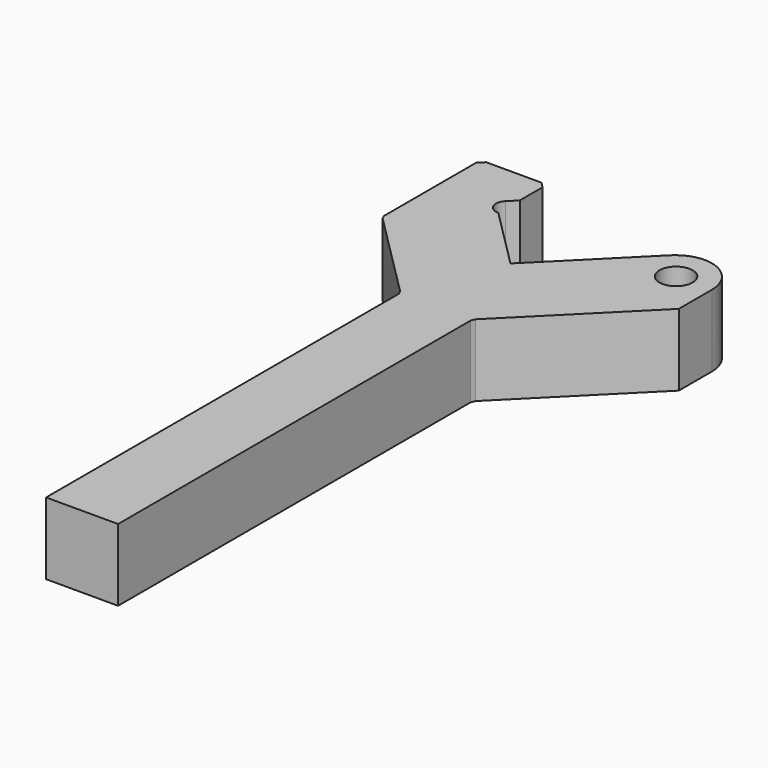
from build123d import *

# Parameters (mm, degrees)
F0_R        = 3
F1_DEPTH    = 13
F2_R        = 7
F3_R        = 6.5
F4_T1_DEPTH = 13
F4_T3_DEPTH = 18.1433659759
F4_T5_DEPTH = 15.2571417204


# Not quite as in the source:
# - a fillet or chamfer that OpenCascade refuses, or shapes differently, is made with other operations: its cross-section is extruded or revolved along the edge and cut away or added


with BuildPart() as f1:
    # F0 (on Top) → F1 (new body)
    with BuildSketch(Plane.XY):
        with BuildLine():
            Line((18, 18), (0, 0))
            Line((0, 0), (-11, 11))
            ThreePointArc((-11, 11), (-12.8659446975, 12.2241130817), (-12.4367385267, 14.4140867148))
            Line((-12.4367385267, 14.4140867148), (-11, 15.8508252416))
            Line((-11, 15.8508252416), (-11, 21.9997463049))
            Line((-11, 21.9997463049), (-23, 21.9997463049))
            Line((-23, 21.9997463049), (-23, -0.1923881554))
            Line((-23, -0.1923881554), (-6.5, -16.6923881554))
            Line((-6.5, -16.6923881554), (-6.5, -96.6923881554))
            Line((-6.5, -96.6923881554), (6.5, -96.6923881554))
            Line((6.5, -96.6923881554), (6.5, -16.6923881554))
            Line((6.5, -16.6923881554), (27.1923881554, 4))
            Line((27.1923881554, 4), (27.1923881554, 18))
            Line((27.1923881554, 18), (18, 18))
        make_face()
        with Locations((20.6923881554, 11.5)):
            Circle(F0_R, mode=Mode.SUBTRACT)
    extrude(amount=F1_DEPTH)

    # F2
    f2_edges = [f1.edges().sort_by_distance(p)[0] for p in [
        (18, 18, 6.5),
    ]]
    fillet(f2_edges, radius=F2_R)

    # F3
    f3_edges = [f1.edges().sort_by_distance(p)[0] for p in [
        (27.192388, 18, 6.5),
    ]]
    fillet(f3_edges, radius=F3_R)

    # F4: chamfer of 1 on 5 edges, made by hand

    # F4_s2 → F4_t1 (join)
    with BuildSketch(Plane.XY):
        Polygon((-6.5, -17.1066017178), (-6.7928932188, -16.3994949366), (-6.5, -16.6923881554), align=None)
        Polygon((6.7928932188, -16.3994949366), (6.5, -17.1066017178), (6.5, -16.6923881554), align=None)
    extrude(amount=F4_T1_DEPTH)

    # F4_s4 → F4_t3 (cut)
    with BuildSketch(Plane.XY.offset(-2.571682988)):
        Polygon((-11, 20.9997463049), (-12, 21.9997463049), (-11, 21.9997463049), align=None)
        Polygon((-22, 21.9997463049), (-23, 20.9997463049), (-23, 21.9997463049), align=None)
    extrude(amount=F4_T3_DEPTH, mode=Mode.SUBTRACT)

    # F4_s6 → F4_t5 (cut)
    with BuildSketch(Plane.XY.offset(-1.1285708602)):
        Polygon((-22.7071067812, -0.4852813742), (-23, 0.2218254069), (-23, -0.1923881554), align=None)
    extrude(amount=F4_T5_DEPTH, mode=Mode.SUBTRACT)


solid = f1.part
